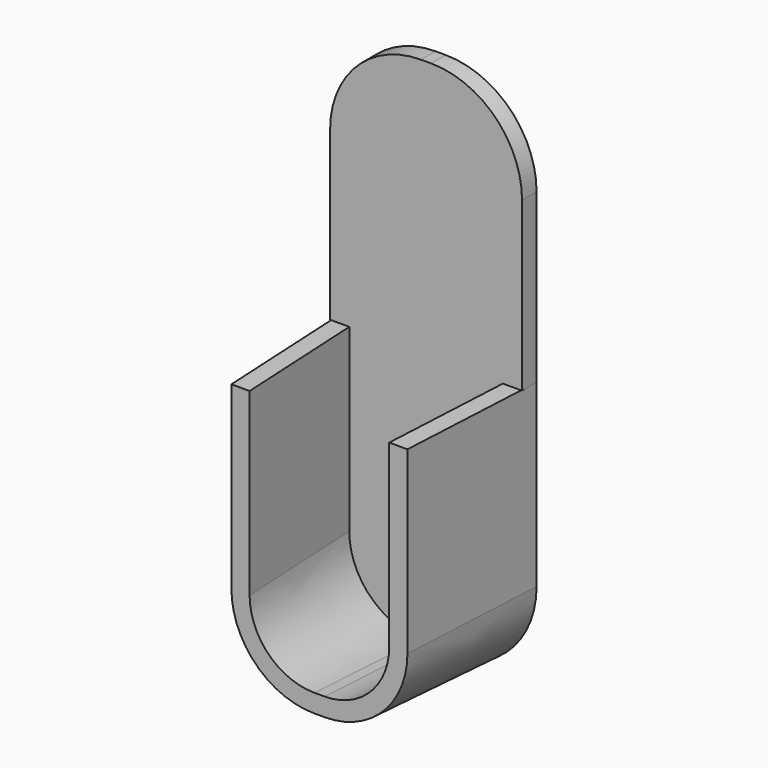
from build123d import *

# Parameters (mm, degrees)
F1_DEPTH = 15
F1_TAPER = 3.0006
F2_T     = -1.8
F3_W     = 16.786262393
F3_H     = 17.0369902626
F4_DEPTH = 28
F6_DEPTH = 1.8


# Not quite as in the source:
# - ends of sketch curves that miss each other by under 0.0002 mm in the source are joined


with BuildPart() as f1:
    # F0 (on Front) → F1 (new body)
    with BuildSketch(Plane.XZ):
        with BuildLine():
            Line((0.5, 19.5), (-0.5, 19.5))
            ThreePointArc((-0.5, 19.5), (-6.8639610307, 16.8639610307), (-9.5, 10.5))
            Line((-9.5, 10.5), (-9.5, -10.5))
            ThreePointArc((-9.5, -10.5), (-6.8639610307, -16.8639610307), (-0.5, -19.5))
            Line((-0.5, -19.5), (0.5, -19.5))
            ThreePointArc((0.5, -19.5), (6.8639610307, -16.8639610307), (9.5, -10.5))
            Line((9.5, -10.5), (9.5, 10.5))
            ThreePointArc((9.5, 10.5), (6.8639610307, 16.8639610307), (0.5, 19.5))
        make_face()
    extrude(amount=F1_DEPTH, taper=F1_TAPER)

    # F2
    f2_openings = [f1.faces().sort_by_distance(p)[0] for p in [
        (0, 0, 0),
        (0, -15, 0),
    ]]
    offset(amount=F2_T, openings=f2_openings)

    # F3 (on Right) → F4 (cut, symmetric)
    with BuildSketch(Plane.YZ):
        with Locations((-8.3931311965, 15.8226261847)):
            Rectangle(F3_W, F3_H)
    extrude(amount=F4_DEPTH, both=True, mode=Mode.SUBTRACT)

    # F5 (on face) → F6 (join)
    with BuildSketch(Plane(origin=(0, 0, 0), x_dir=(-1, 0, 0), z_dir=(0, 1, 0))):
        with BuildLine():
            Line((0.5000003055, 32.8999999631), (-0.4999996945, 32.8999999631))
            ThreePointArc((-0.4999996945, 32.8999999631), (-6.8639607252, 30.2639609938), (-9.4999996945, 23.8999999631))
            Line((-9.4999996945, 23.8999999631), (-9.4999998419, 7.3041310534))
            Line((-9.4999998419, 7.3041310534), (-7.6975287879, 7.3041310534))
            Line((-7.6975287879, 7.3041310534), (-7.6975287879, -10.5))
            ThreePointArc((-7.6975287879, -10.5), (-5.5894214137, -15.5894214137), (-0.5, -17.6975287879))
            Line((-0.5, -17.6975287879), (0.5, -17.6975287879))
            ThreePointArc((0.5, -17.6975287879), (5.5894214137, -15.5894214137), (7.6975287879, -10.5))
            Line((7.6975287879, -10.5), (7.6975287879, 7.3041310534))
            Line((7.6975287879, 7.3041310534), (9.5, 7.3041310534))
            Line((9.5, 7.3041310534), (9.5000003055, 23.8999999631))
            ThreePointArc((9.5000003055, 23.8999999631), (6.8639613362, 30.2639609938), (0.5000003055, 32.8999999631))
        make_face()
    extrude(amount=-F6_DEPTH)


solid = f1.part
